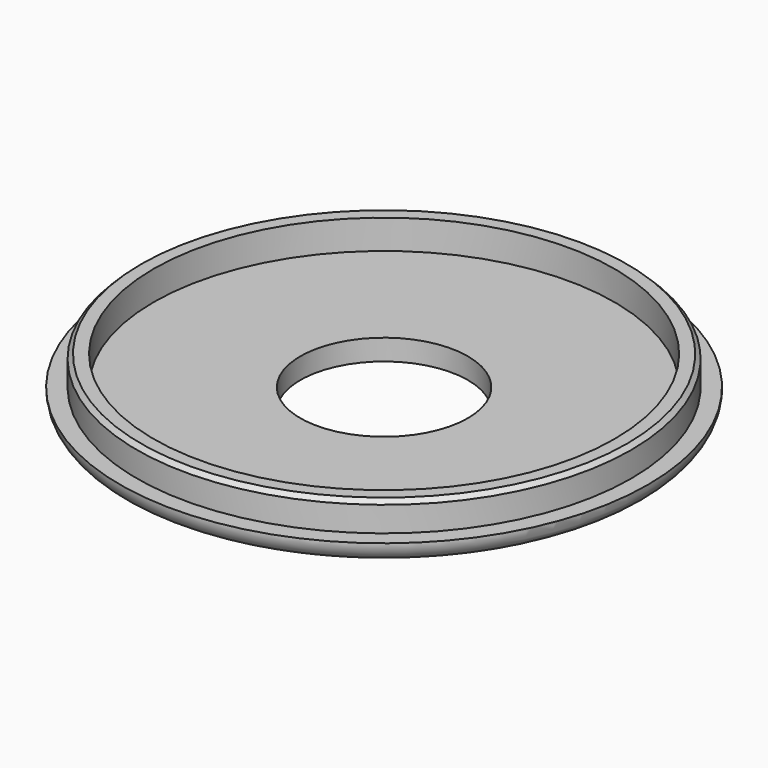
from build123d import *

# Parameters (mm, degrees)
F0_R     = 59
F0_R_2   = 55
F1_DEPTH = 7
F0_R_3   = 63
F0_R_4   = 20
F2_DEPTH = 5
F3_R     = 4.99999
F4_SIZE  = 1


# Not quite as in the source:
# - a fillet or chamfer is up to 0.001 mm smaller than in the source, because OpenCascade refuses the exact size


with BuildPart() as f1:
    # F0 (on Top) → F1 (new body)
    with BuildSketch(Plane.XY):
        Circle(F0_R)
        Circle(F0_R_2, mode=Mode.SUBTRACT)
    extrude(amount=F1_DEPTH)

    # F0 (on Top) → F2 (join)
    with BuildSketch(Plane.XY):
        Circle(F0_R_3)
        Circle(F0_R, mode=Mode.SUBTRACT)
        Circle(F0_R)
        Circle(F0_R_2, mode=Mode.SUBTRACT)
        Circle(F0_R_2)
        Circle(F0_R_4, mode=Mode.SUBTRACT)
    extrude(amount=-F2_DEPTH)

    # F3 (radius 5 in the source; OpenCascade refuses exactly that, so slightly less here)
    f3_edges = [f1.edges().sort_by_distance(p)[0] for p in [
        (-63, 0, -5),
    ]]
    fillet(f3_edges, radius=F3_R)

    # F4
    f4_edges = [f1.edges().sort_by_distance(p)[0] for p in [
        (-59, 0, 7),
    ]]
    chamfer(f4_edges, length=F4_SIZE)


solid = f1.part
